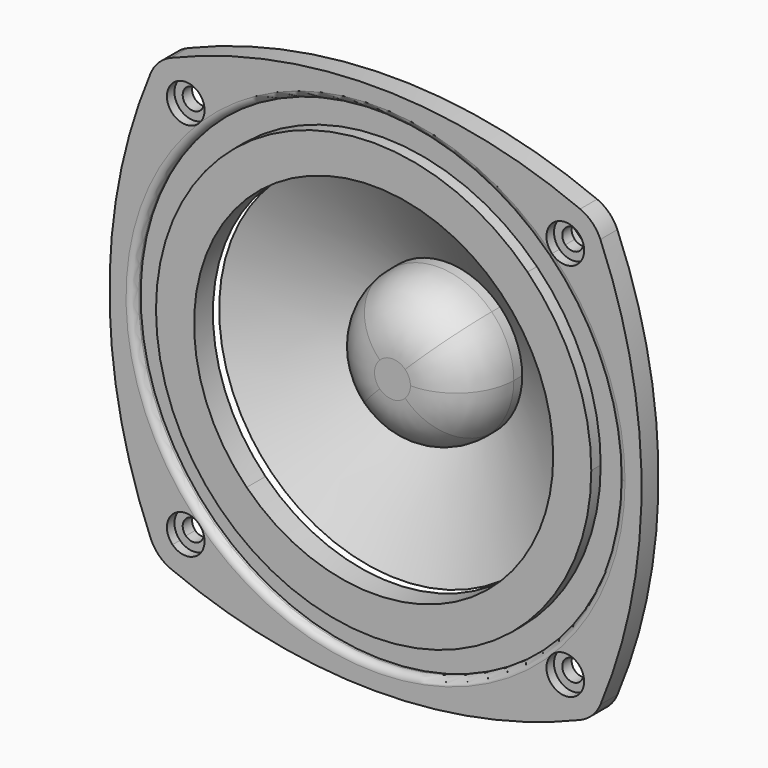
from build123d import *

# Parameters (mm, degrees)
F1_DEPTH = 4.5
F2_R     = 1.49999
F3_DEPTH = 4.5
F4_DEPTH = 2.5
F5_DEPTH = 5
F6_DEPTH = 20
F8_DEPTH = 20
F9_DEPTH = 2.5
F10_R    = 12.2
F11_R    = 8


# Not quite as in the source:
# - a fillet or chamfer that OpenCascade refuses, or shapes differently, is made with other operations: its cross-section is extruded or revolved along the edge and cut away or added
# - a fillet or chamfer is up to 0.001 mm smaller than in the source, because OpenCascade refuses the exact size
# - a feature names something its author has since deleted; it is built from what else it names


with BuildPart() as f1:
    # F0 (on Front) → F1 (new body)
    with BuildSketch(Plane.XZ):
        with BuildLine():
            ThreePointArc((-36.418497781, 36.4135005098), (-0.0069910873, 51.4999995255), (36.4086102268, 36.4233867365))
            Line((36.4086102268, 36.4233867365), (37.4690661738, 37.4842730718))
            ThreePointArc((37.4690661738, 37.4842730718), (37.4760856161, 43.1329397491), (43.1247489801, 43.1422512486))
            Line((43.1247489801, 43.1422512486), (46.4569826347, 46.4758372971))
            ThreePointArc((46.4569826347, 46.4758372971), (-0.0070362771, 56.5000696821), (-46.4677732762, 46.460637136))
            Line((-46.4677732762, 46.460637136), (-43.1367254099, 43.1302982437))
            ThreePointArc((-43.1367254099, 43.1302982437), (-38.7764524198, 44.0014736508), (-36.3050865276, 40.3050865276))
            ThreePointArc((-36.3050865276, 40.3050865276), (-36.6102754643, 38.772646902), (-37.4792721307, 37.4740490863))
            Line((-37.4792721307, 37.4740490863), (-36.418497781, 36.4135005098))
        make_face()
        with BuildLine():
            ThreePointArc((-36.4086102268, -36.4233867365), (-51.4999995255, -0.0069910873), (-36.418497781, 36.4135005098))
            Line((-36.418497781, 36.4135005098), (-37.4792721307, 37.4740490863))
            ThreePointArc((-37.4792721307, 37.4740490863), (-43.1332126057, 37.4763583883), (-43.1367254099, 43.1302982437))
            Line((-43.1367254099, 43.1302982437), (-46.4677732762, 46.460637136))
            ThreePointArc((-46.4677732762, 46.460637136), (-46.4718053226, 46.4588099646), (-46.4758372971, 46.4569826347))
            ThreePointArc((-46.4758372971, 46.4569826347), (-56.4999982578, -0.0114629944), (-46.4569826347, -46.4758372971))
            Line((-46.4569826347, -46.4758372971), (-43.1247489801, -43.1422512486))
            ThreePointArc((-43.1247489801, -43.1422512486), (-43.1340874392, -37.4772333061), (-37.4690661738, -37.4842730718))
            Line((-37.4690661738, -37.4842730718), (-36.4086102268, -36.4233867365))
        make_face()
        with BuildLine():
            Line((37.4820302823, -37.4712987029), (36.4212517549, -36.4107459496))
            ThreePointArc((36.4212517549, -36.4107459496), (0.0089386482, -51.4999992243), (-36.4086102268, -36.4233867365))
            Line((-36.4086102268, -36.4233867365), (-37.4690661738, -37.4842730718))
            ThreePointArc((-37.4690661738, -37.4842730718), (-36.6075142555, -38.7793213778), (-36.3050865276, -40.3050865276))
            ThreePointArc((-36.3050865276, -40.3050865276), (-38.7686376691, -43.9982321929), (-43.1247489801, -43.1422512486))
            Line((-43.1247489801, -43.1422512486), (-46.4569826347, -46.4758372971))
            ThreePointArc((-46.4569826347, -46.4758372971), (-23.752139626, -53.9690179835), (0.0228922165, -56.4999296251))
            ThreePointArc((0.0228922165, -56.4999296251), (23.7828730619, -53.9574018264), (46.4714717713, -46.4588268959))
            Line((46.4714717713, -46.4588268959), (43.1394752061, -43.1275395067))
            ThreePointArc((43.1394752061, -43.1275395067), (37.4769604495, -43.133814667), (37.4820302823, -37.4712987029))
        make_face()
        with BuildLine():
            ThreePointArc((36.4086102268, 36.4233867365), (47.5777964322, 19.7130232755), (51.5, 0))
            ThreePointArc((51.5, 0), (47.5812172258, -19.7047650915), (36.4212517549, -36.4107459496))
            Line((36.4212517549, -36.4107459496), (37.4820302823, -37.4712987029))
            ThreePointArc((37.4820302823, -37.4712987029), (41.8393249411, -36.611022033), (44.3050865276, -40.3050865276))
            ThreePointArc((44.3050865276, -40.3050865276), (44.0022174906, -41.8319207174), (43.1394752061, -43.1275395067))
            Line((43.1394752061, -43.1275395067), (46.4714717713, -46.4588268959))
            ThreePointArc((46.4714717713, -46.4588268959), (46.4736545447, -46.4578376778), (46.4758372971, -46.4568484132))
            ThreePointArc((46.4758372971, -46.4568484132), (56.499998251, 0.0115301081), (46.4569826347, 46.4758372971))
            Line((46.4569826347, 46.4758372971), (43.1247489801, 43.1422512486))
            ThreePointArc((43.1247489801, 43.1422512486), (43.9982321929, 41.8415353862), (44.3050865276, 40.3050865276))
            ThreePointArc((44.3050865276, 40.3050865276), (41.8308516774, 36.6075142555), (37.4690661738, 37.4842730718))
            Line((37.4690661738, 37.4842730718), (36.4086102268, 36.4233867365))
        make_face()
    extrude(amount=F1_DEPTH)

    # F2 (radius 1.5 in the source; OpenCascade refuses exactly that, so slightly less here)
    f2_edges = [f1.edges().sort_by_distance(p)[0] for p in [
        (-36.40861, -4.5, -36.423387),
    ]]
    fillet(f2_edges, radius=F2_R)

    # F11
    f11_edges = [f1.edges().sort_by_distance(p)[0] for p in [
        (-46.475837, -2.25, 46.456983),
        (46.456983, -2.25, 46.475837),
        (46.475837, -2.25, -46.456848),
        (-46.456983, -2.25, -46.475837),
    ]]
    fillet(f11_edges, radius=F11_R)


with BuildPart() as f3:
    # F0 (on Front) → F3 (new body)
    with BuildSketch(Plane.XZ):
        with BuildLine():
            Line((32.6815175192, 32.6947813806), (36.4086102268, 36.4233867365))
            ThreePointArc((36.4086102268, 36.4233867365), (-0.0069910873, 51.4999995255), (-36.418497781, 36.4135005098))
            Line((-36.418497781, 36.4135005098), (-32.6902519342, 32.686048176))
            ThreePointArc((-32.6902519342, 32.686048176), (-0.0061757362, 46.2280248198), (32.6815175192, 32.6947813806))
        make_face()
        with BuildLine():
            Line((-32.6902519342, 32.686048176), (-36.418497781, 36.4135005098))
            ThreePointArc((-36.418497781, 36.4135005098), (-51.4999995255, -0.0069910873), (-36.4086102268, -36.4233867365))
            Line((-36.4086102268, -36.4233867365), (-32.6815175192, -32.6947813806))
            ThreePointArc((-32.6815175192, -32.6947813806), (-46.2280248198, -0.0061757362), (-32.6902519342, 32.686048176))
        make_face()
        with BuildLine():
            ThreePointArc((-36.4086102268, -36.4233867365), (0.0089386482, -51.4999992243), (36.4212517549, -36.4107459496))
            Line((36.4212517549, -36.4107459496), (32.6930059081, -32.6832936158))
            ThreePointArc((32.6930059081, -32.6832936158), (0.0081232971, -46.2280245186), (-32.6815175192, -32.6947813806))
            Line((-32.6815175192, -32.6947813806), (-36.4086102268, -36.4233867365))
        make_face()
        with BuildLine():
            ThreePointArc((36.4212517549, -36.4107459496), (47.5812172258, -19.7047650915), (51.5, 0))
            ThreePointArc((51.5, 0), (47.5777964322, 19.7130232755), (36.4086102268, 36.4233867365))
            Line((36.4086102268, 36.4233867365), (32.6815175192, 32.6947813806))
            ThreePointArc((32.6815175192, 32.6947813806), (42.7073315333, 17.6950317939), (46.2280252324, 0))
            ThreePointArc((46.2280252324, 0), (42.7104402865, -17.6875268882), (32.6930059081, -32.6832936158))
            Line((32.6930059081, -32.6832936158), (36.4212517549, -36.4107459496))
        make_face()
    extrude(amount=-F3_DEPTH)


with BuildPart() as f4:
    # F0 (on Front) → F4 (new body)
    with BuildSketch(Plane.XZ):
        with BuildLine():
            ThreePointArc((36.4212517549, -36.4107459496), (47.5812172258, -19.7047650915), (51.5, 0))
            ThreePointArc((51.5, 0), (47.5777964322, 19.7130232755), (36.4086102268, 36.4233867365))
            Line((36.4086102268, 36.4233867365), (32.6815175192, 32.6947813806))
            ThreePointArc((32.6815175192, 32.6947813806), (42.7073315333, 17.6950317939), (46.2280252324, 0))
            ThreePointArc((46.2280252324, 0), (42.7104402865, -17.6875268882), (32.6930059081, -32.6832936158))
            Line((32.6930059081, -32.6832936158), (36.4212517549, -36.4107459496))
        make_face()
        with BuildLine():
            Line((32.6815175192, 32.6947813806), (36.4086102268, 36.4233867365))
            ThreePointArc((36.4086102268, 36.4233867365), (-0.0069910873, 51.4999995255), (-36.418497781, 36.4135005098))
            Line((-36.418497781, 36.4135005098), (-32.6902519342, 32.686048176))
            ThreePointArc((-32.6902519342, 32.686048176), (-0.0061757362, 46.2280248198), (32.6815175192, 32.6947813806))
        make_face()
        with BuildLine():
            ThreePointArc((-36.4086102268, -36.4233867365), (0.0089386482, -51.4999992243), (36.4212517549, -36.4107459496))
            Line((36.4212517549, -36.4107459496), (32.6930059081, -32.6832936158))
            ThreePointArc((32.6930059081, -32.6832936158), (0.0081232971, -46.2280245186), (-32.6815175192, -32.6947813806))
            Line((-32.6815175192, -32.6947813806), (-36.4086102268, -36.4233867365))
        make_face()
        with BuildLine():
            Line((-32.6902519342, 32.686048176), (-36.418497781, 36.4135005098))
            ThreePointArc((-36.418497781, 36.4135005098), (-51.4999995255, -0.0069910873), (-36.4086102268, -36.4233867365))
            Line((-36.4086102268, -36.4233867365), (-32.6815175192, -32.6947813806))
            ThreePointArc((-32.6815175192, -32.6947813806), (-46.2280248198, -0.0061757362), (-32.6902519342, 32.686048176))
        make_face()
    extrude(amount=F4_DEPTH)

    # F0 (on Front) → F5 (join)
    with BuildSketch(Plane.XZ):
        with BuildLine():
            Line((26.9640777334, 26.9750211601), (32.6815175192, 32.6947813806))
            ThreePointArc((32.6815175192, 32.6947813806), (-0.0061757362, 46.2280248198), (-32.6902519342, 32.686048176))
            Line((-32.6902519342, 32.686048176), (-26.9710432067, 26.9680567142))
            ThreePointArc((-26.9710432067, 26.9680567142), (-0.0049249702, 38.1407030657), (26.9640777334, 26.9750211601))
        make_face()
        with BuildLine():
            Line((-26.9710432067, 26.9680567142), (-32.6902519342, 32.686048176))
            ThreePointArc((-32.6902519342, 32.686048176), (-46.2280248198, -0.0061757362), (-32.6815175192, -32.6947813806))
            Line((-32.6815175192, -32.6947813806), (-26.9640777334, -26.9750211601))
            ThreePointArc((-26.9640777334, -26.9750211601), (-38.1407030657, -0.0049249702), (-26.9710432067, 26.9680567142))
        make_face()
        with BuildLine():
            ThreePointArc((-32.6815175192, -32.6947813806), (0.0081232971, -46.2280245186), (32.6930059081, -32.6832936158))
            Line((32.6930059081, -32.6832936158), (26.9737971806, -26.965302154))
            ThreePointArc((26.9737971806, -26.965302154), (0.0068725311, -38.1407027645), (-26.9640777334, -26.9750211601))
            Line((-26.9640777334, -26.9750211601), (-32.6815175192, -32.6947813806))
        make_face()
        with BuildLine():
            ThreePointArc((46.2280252324, 0), (42.7073315333, 17.6950317939), (32.6815175192, 32.6947813806))
            Line((32.6815175192, 32.6947813806), (26.9640777334, 26.9750211601))
            ThreePointArc((26.9640777334, 26.9750211601), (35.2359343954, 14.5993897776), (38.1407033836, 0))
            ThreePointArc((38.1407033836, 0), (35.2385644713, -14.5930404166), (26.9737971806, -26.965302154))
            Line((26.9737971806, -26.965302154), (32.6930059081, -32.6832936158))
            ThreePointArc((32.6930059081, -32.6832936158), (42.7104402865, -17.6875268882), (46.2280252324, 0))
        make_face()
    extrude(amount=F5_DEPTH)


with BuildPart() as f4b:
    # F0 (on Front) → F4, piece 2 (new body)
    with BuildSketch(Plane.XZ):
        with BuildLine():
            Line((38.719603259, -38.7086082769), (37.4820302823, -37.4712987029))
            ThreePointArc((37.4820302823, -37.4712987029), (37.4769604495, -43.133814667), (43.1394752061, -43.1275395067))
            Line((43.1394752061, -43.1275395067), (41.9019022294, -41.8902299327))
            ThreePointArc((41.9019022294, -41.8902299327), (38.7142656087, -41.896246106), (38.719603259, -38.7086082769))
        make_face()
        with BuildLine():
            ThreePointArc((44.3050865276, -40.3050865276), (41.8393249411, -36.611022033), (37.4820302823, -37.4712987029))
            Line((37.4820302823, -37.4712987029), (38.719603259, -38.7086082769))
            ThreePointArc((38.719603259, -38.7086082769), (41.1697143799, -38.2278482945), (42.5550865276, -40.3050865276))
            ThreePointArc((42.5550865276, -40.3050865276), (42.3853912324, -41.1623101481), (41.9019022294, -41.8902299327))
            Line((41.9019022294, -41.8902299327), (43.1394752061, -43.1275395067))
            ThreePointArc((43.1394752061, -43.1275395067), (44.0022174906, -41.8319207174), (44.3050865276, -40.3050865276))
        make_face()
    extrude(amount=F4_DEPTH)


with BuildPart() as f4c:
    # F0 (on Front) → F4, piece 3 (new body)
    with BuildSketch(Plane.XZ):
        with BuildLine():
            Line((-38.7168418581, 38.7113554117), (-37.4792721307, 37.4740490863))
            ThreePointArc((-37.4792721307, 37.4740490863), (-36.6102754643, 38.772646902), (-36.3050865276, 40.3050865276))
            ThreePointArc((-36.3050865276, 40.3050865276), (-38.7764524198, 44.0014736508), (-43.1367254099, 43.1302982437))
            Line((-43.1367254099, 43.1302982437), (-41.8991556824, 41.8929919183))
            ThreePointArc((-41.8991556824, 41.8929919183), (-39.4460625461, 42.3846484525), (-38.0550865276, 40.3050865276))
            ThreePointArc((-38.0550865276, 40.3050865276), (-38.2271006631, 39.4422570272), (-38.7168418581, 38.7113554117))
        make_face()
        with BuildLine():
            ThreePointArc((-43.1367254099, 43.1302982437), (-43.1332126057, 37.4763583883), (-37.4792721307, 37.4740490863))
            Line((-37.4792721307, 37.4740490863), (-38.7168418581, 38.7113554117))
            ThreePointArc((-38.7168418581, 38.7113554117), (-41.8959074466, 38.7139269493), (-41.8991556824, 41.8929919183))
            Line((-41.8991556824, 41.8929919183), (-43.1367254099, 43.1302982437))
        make_face()
    extrude(amount=F4_DEPTH)


with BuildPart() as f6:
    # F0 (on Front) → F6 (new body)
    with BuildSketch(Plane.XZ):
        with BuildLine():
            Line((11.3179053137, 11.322498709), (26.9640777334, 26.9750211601))
            ThreePointArc((26.9640777334, 26.9750211601), (-0.0049249702, 38.1407030657), (-26.9710432067, 26.9680567142))
            Line((-26.9710432067, 26.9680567142), (-11.3200299168, 11.3203745567))
            ThreePointArc((-11.3200299168, 11.3203745567), (-0.0015021619, 16.009203119), (11.3179053137, 11.322498709))
        make_face()
        with BuildLine():
            Line((-11.3200299168, 11.3203745567), (-26.9710432067, 26.9680567142))
            ThreePointArc((-26.9710432067, 26.9680567142), (-38.1407030657, -0.0049249702), (-26.9640777334, -26.9750211601))
            Line((-26.9640777334, -26.9750211601), (-11.317838203, -11.322431571))
            ThreePointArc((-11.317838203, -11.322431571), (-16.0091360037, -0.001482496), (-11.3200299168, 11.3203745567))
        make_face()
        with BuildLine():
            ThreePointArc((-26.9640777334, -26.9750211601), (0.0068725311, -38.1407027645), (26.9737971806, -26.965302154))
            Line((26.9737971806, -26.965302154), (11.32271678, -11.3175529001))
            ThreePointArc((11.32271678, -11.3175529001), (0.0034497081, -16.0090685963), (-11.317838203, -11.322431571))
            Line((-11.317838203, -11.322431571), (-26.9640777334, -26.9750211601))
        make_face()
        with BuildLine():
            ThreePointArc((38.1407033836, 0), (35.2359343954, 14.5993897776), (26.9640777334, 26.9750211601))
            Line((26.9640777334, 26.9750211601), (11.3179053137, 11.322498709))
            ThreePointArc((11.3179053137, 11.322498709), (14.7899006806, 6.1279766929), (16.0091360787, 6.71107e-05))
            ThreePointArc((16.0091360787, 6.71107e-05), (14.7912026505, -6.1246991818), (11.32271678, -11.3175529001))
            Line((11.32271678, -11.3175529001), (26.9737971806, -26.965302154))
            ThreePointArc((26.9737971806, -26.965302154), (35.2385644713, -14.5930404166), (38.1407033836, 0))
        make_face()
    extrude(amount=-F6_DEPTH)

    # F7: chamfer of 25 x 14.4337567297 on 1 edges, made by hand

    # F7_s1 → F7_t2 (revolve, cut)
    with BuildSketch(Plane(origin=(-3.35554e-05, 0, 3.3542e-05), x_dir=(0, 1, 0), z_dir=(-0.7072481327, 0, 0.7069654014))):
        Polygon((14.4337567297, -16.0091835427), (0, -41.0091835427), (0, -16.0091835427), align=None)
    revolve(axis=Axis((0, 0, 6.71107e-05), (0, 1, 0)), mode=Mode.SUBTRACT)


with BuildPart() as f8:
    # F0 (on Front) → F8 (new body)
    with BuildSketch(Plane.XZ):
        with BuildLine():
            Line((0.0013768541, 0.0013774129), (11.3179053137, 11.322498709))
            ThreePointArc((11.3179053137, 11.322498709), (-0.0015021619, 16.009203119), (-11.3200299168, 11.3203745567))
            Line((-11.3200299168, 11.3203745567), (0.0013768541, 0.0013774129))
        make_face()
        with BuildLine():
            Line((0.0013768541, 0.0013774129), (-11.3200299168, 11.3203745567))
            ThreePointArc((-11.3200299168, 11.3203745567), (-16.0091360037, -0.001482496), (-11.317838203, -11.322431571))
            Line((-11.317838203, -11.322431571), (0.0013768541, 0.0013774129))
        make_face()
        with BuildLine():
            ThreePointArc((-11.317838203, -11.322431571), (0.0034497081, -16.0090685963), (11.32271678, -11.3175529001))
            Line((11.32271678, -11.3175529001), (0.002690971, 6.35758e-05))
            Line((0.002690971, 6.35758e-05), (0.0013768541, 0.0013774129))
            Line((0.0013768541, 0.0013774129), (-11.317838203, -11.322431571))
        make_face()
        with BuildLine():
            ThreePointArc((16.0091360787, 6.71107e-05), (14.7899006806, 6.1279766929), (11.3179053137, 11.322498709))
            Line((11.3179053137, 11.322498709), (0.0013768541, 0.0013774129))
            Line((0.0013768541, 0.0013774129), (0.002690971, 6.35758e-05))
            Line((0.002690971, 6.35758e-05), (11.32271678, -11.3175529001))
            ThreePointArc((11.32271678, -11.3175529001), (14.7912026505, -6.1246991818), (16.0091360787, 6.71107e-05))
        make_face()
    extrude(amount=-F8_DEPTH)

    # F10
    f10_edges = [f8.edges().sort_by_distance(p)[0] for p in [
        (-11.317905, 0, -11.322364),
    ]]
    fillet(f10_edges, radius=F10_R)


with BuildPart() as f9:
    # F0 (on Front) → F9 (new body)
    with BuildSketch(Plane.XZ):
        with BuildLine():
            ThreePointArc((43.1247489801, 43.1422512486), (37.4760856161, 43.1329397491), (37.4690661738, 37.4842730718))
            Line((37.4690661738, 37.4842730718), (38.7062611504, 38.7219701665))
            ThreePointArc((38.7062611504, 38.7219701665), (38.7137735149, 41.8957539647), (41.8875540036, 41.9045541539))
            Line((41.8875540036, 41.9045541539), (43.1247489801, 43.1422512486))
        make_face()
        with BuildLine():
            Line((38.7062611504, 38.7219701665), (37.4690661738, 37.4842730718))
            ThreePointArc((37.4690661738, 37.4842730718), (41.8308516774, 36.6075142555), (44.3050865276, 40.3050865276))
            ThreePointArc((44.3050865276, 40.3050865276), (43.9982321929, 41.8415353862), (43.1247489801, 43.1422512486))
            Line((43.1247489801, 43.1422512486), (41.8875540036, 41.9045541539))
            ThreePointArc((41.8875540036, 41.9045541539), (42.3815079469, 41.1716741398), (42.5550865276, 40.3050865276))
            ThreePointArc((42.5550865276, 40.3050865276), (41.1609904069, 38.2242384915), (38.7062611504, 38.7219701665))
        make_face()
    extrude(amount=F9_DEPTH)


with BuildPart() as f9b:
    # F0 (on Front) → F9, piece 2 (new body)
    with BuildSketch(Plane.XZ):
        with BuildLine():
            Line((-38.7062611504, -38.7219701665), (-37.4690661738, -37.4842730718))
            ThreePointArc((-37.4690661738, -37.4842730718), (-43.1340874392, -37.4772333061), (-43.1247489801, -43.1422512486))
            Line((-43.1247489801, -43.1422512486), (-41.8875540036, -41.9045541539))
            ThreePointArc((-41.8875540036, -41.9045541539), (-41.8963995404, -38.7144190905), (-38.7062611504, -38.7219701665))
        make_face()
        with BuildLine():
            ThreePointArc((-36.3050865276, -40.3050865276), (-36.6075142555, -38.7793213778), (-37.4690661738, -37.4842730718))
            Line((-37.4690661738, -37.4842730718), (-38.7062611504, -38.7219701665))
            ThreePointArc((-38.7062611504, -38.7219701665), (-38.2242384915, -39.4491826483), (-38.0550865276, -40.3050865276))
            ThreePointArc((-38.0550865276, -40.3050865276), (-39.4384989155, -42.3815079469), (-41.8875540036, -41.9045541539))
            Line((-41.8875540036, -41.9045541539), (-43.1247489801, -43.1422512486))
            ThreePointArc((-43.1247489801, -43.1422512486), (-38.7686376691, -43.9982321929), (-36.3050865276, -40.3050865276))
        make_face()
    extrude(amount=F9_DEPTH)


solid = Compound([f1.part, f3.part, f4.part, f4b.part, f4c.part, f6.part, f8.part, f9.part, f9b.part])
